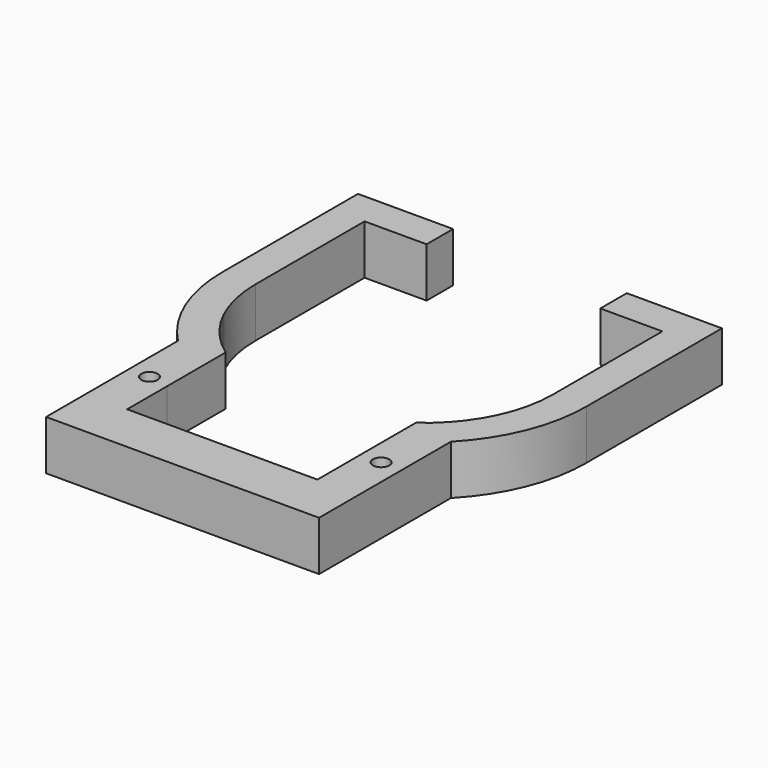
from build123d import *

# Parameters (mm, degrees)
F0_R     = 1
F0_W     = 23
F0_H     = 6
F1_DEPTH = 6


# Not quite as in the source:
# - a feature names something its author has since deleted; it is built from what else it names


with BuildPart() as f1:
    # F0 (on Top) → F1 (new body)
    with BuildSketch(Plane.XY):
        with BuildLine():
            Line((-16.5, -21.0738723458), (-16.5, -14.1520673478))
            ThreePointArc((-16.5, -14.1520673478), (-17.620350525, -10.9095454242), (-18, -7.5))
            Line((-18, -7.5), (-18, 9))
            Line((-18, 9), (-10.5, 9))
            Line((-10.5, 9), (-10.5, 13.0000002682))
            Line((-10.5, 13.0000002682), (-22.0000002682, 13.0000002682))
            Line((-22.0000002682, 13.0000002682), (-22.0000002682, -7.5))
            ThreePointArc((-22.0000002682, -7.5), (-20.5727697686, -14.8229094869), (-16.5, -21.0738723458))
        make_face()
        with BuildLine():
            Line((14.3321600082, -23), (11.4999999106, -23))
            Line((11.5, -23), (11.5, -24.7988442176))
            ThreePointArc((11.4999999553, -24.7988442176), (12.9548401383, -23.9604473859), (14.3321600082, -23))
        make_face()
        with BuildLine():
            ThreePointArc((14.3321600082, -23), (12.9548401383, -23.9604473859), (11.4999999553, -24.7988442176))
            Line((11.5, -24.7988442176), (11.5, -29))
            Line((11.4999999106, -29), (11.4999999106, -35))
            Line((11.4999999106, -35), (11.4999999106, -41))
            Line((11.4999999106, -41), (16.4999999106, -41))
            Line((16.4999999106, -41), (16.4999999106, -23))
            Line((16.4999999106, -23), (14.3321600082, -23))
        make_face()
        with Locations((14, -28.5)):
            Circle(F0_R, mode=Mode.SUBTRACT)
        with BuildLine():
            ThreePointArc((18, -7.5), (17.620350525, -10.9095454242), (16.5, -14.1520673478))
            Line((16.5, -14.1520673478), (16.5, -21.0738723458))
            ThreePointArc((16.5, -21.0738723458), (20.5727697686, -14.8229094869), (22.0000002682, -7.5))
            Line((22.0000002682, -7.5), (22.0000002682, 13.0000002682))
            Line((22.0000002682, 13.0000002682), (10.5, 13.0000002682))
            Line((10.5, 13.0000002682), (10.5, 9))
            Line((10.5, 9), (18, 9))
            Line((18, 9), (18, -7.5))
        make_face()
        with BuildLine():
            Line((-11.5, -24.7988441711), (-11.5, -23))
            Line((-11.5000000894, -23), (-14.3321600082, -23))
            ThreePointArc((-14.3321600082, -23), (-12.9548401808, -23.9604473589), (-11.5000000447, -24.7988441711))
        make_face()
        with BuildLine():
            Line((-11.5, -29), (-11.5, -24.7988441711))
            ThreePointArc((-11.5000000447, -24.7988441711), (-12.9548401808, -23.9604473589), (-14.3321600082, -23))
            Line((-14.3321600082, -23), (-16.5000000894, -23))
            Line((-16.5000000894, -23), (-16.5000000894, -41))
            Line((-16.5000000894, -41), (-11.5000000894, -41))
            Line((-11.5000000894, -41), (-11.5000000894, -35))
            Line((-11.5000000894, -35), (-11.5000000894, -29))
        make_face()
        with Locations((-14, -28.5)):
            Circle(F0_R, mode=Mode.SUBTRACT)
        with BuildLine():
            Line((-16.5000000894, -23), (-14.3321600082, -23))
            ThreePointArc((-14.3321600082, -23), (-15.4519347824, -22.0772904153), (-16.5, -21.0738723458))
            Line((-16.5, -21.0738723458), (-16.5, -23))
        make_face()
        with Locations((-8.94e-08, -38)):
            Rectangle(F0_W, F0_H)
        with BuildLine():
            ThreePointArc((16.5, -21.0738723458), (15.4519347824, -22.0772904153), (14.3321600082, -23))
            Line((14.3321600082, -23), (16.4999999106, -23))
            Line((16.5, -23), (16.5, -21.0738723458))
        make_face()
        with BuildLine():
            ThreePointArc((16.5, -14.1520673478), (14.3807555592, -17.4547801253), (11.5, -20.1194294641))
            Line((11.5, -20.1194294641), (11.5, -23))
            Line((11.4999999106, -23), (14.3321600082, -23))
            ThreePointArc((14.3321600082, -23), (15.4519347824, -22.0772904153), (16.5, -21.0738723458))
            Line((16.5, -21.0738723458), (16.5, -14.1520673478))
        make_face()
        with BuildLine():
            Line((-11.5, -23), (-11.5, -20.1194294641))
            ThreePointArc((-11.5, -20.1194294641), (-14.3807555592, -17.4547801253), (-16.5, -14.1520673478))
            Line((-16.5, -14.1520673478), (-16.5, -21.0738723458))
            ThreePointArc((-16.5, -21.0738723458), (-15.4519347824, -22.0772904153), (-14.3321600082, -23))
            Line((-14.3321600082, -23), (-11.5000000894, -23))
        make_face()
    extrude(amount=F1_DEPTH)


solid = f1.part
